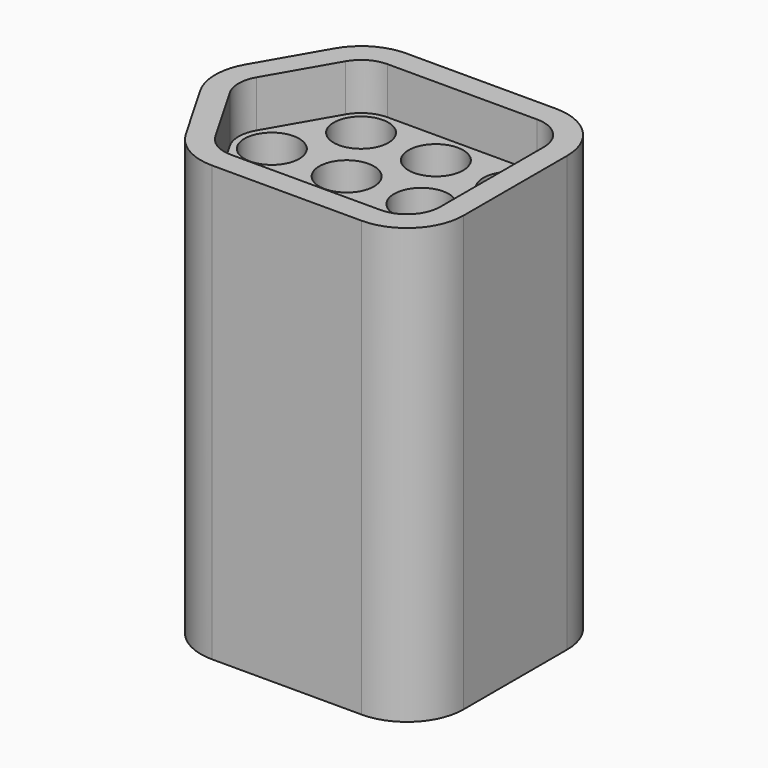
from build123d import *

# Parameters (mm, degrees)
F0_R     = 0.585
F1_DEPTH = 9.3
F2_DEPTH = 1
F3_DEPTH = 8.3
F4_R     = 0.45
F5_DEPTH = 9.301


# Not quite as in the source:
# - a feature names something its author has since deleted; it is built from what else it names


with BuildPart() as f1:
    # F0 (on Top) → F1 (new body)
    with BuildSketch(Plane.XY):
        with BuildLine():
            Line((0, 1.21), (-3.2, 1.21))
            ThreePointArc((-3.2, 1.21), (-3.8050588257, 1.0478567734), (-4.2479586591, 0.6048823429))
            Line((-4.2479586591, 0.6048823429), (-5.0479586591, -0.7811176571))
            ThreePointArc((-5.0479586591, -0.7811176571), (-5.21, -1.386), (-5.0479586591, -1.9908823429))
            Line((-5.0479586591, -1.9908823429), (-4.2479586591, -3.3768823429))
            ThreePointArc((-4.2479586591, -3.3768823429), (-3.8050588257, -3.8198567734), (-3.2, -3.982))
            Line((-3.2, -3.982), (0, -3.982))
            ThreePointArc((0, -3.982), (0.8555992052, -3.6275992052), (1.21, -2.772))
            Line((1.21, -2.772), (1.21, 0))
            ThreePointArc((1.21, 0), (0.8555992052, 0.8555992052), (0, 1.21))
        make_face()
        with BuildLine():
            ThreePointArc((-3.8149178909, 0.3549309616), (-3.5550345175, 0.6148581067), (-3.2, 0.71))
            Line((-3.2, 0.71), (0, 0.71))
            ThreePointArc((0, 0.71), (0.5020458146, 0.5020458146), (0.71, 0))
            Line((0.71, 0), (0.71, -2.772))
            ThreePointArc((0.71, -2.772), (0.5020458146, -3.2740458146), (0, -3.482))
            Line((0, -3.482), (-3.2, -3.482))
            ThreePointArc((-3.2, -3.482), (-3.5550345175, -3.3868581067), (-3.8149178909, -3.1269309616))
            Line((-3.8149178909, -3.1269309616), (-4.6149178909, -1.7409309616))
            ThreePointArc((-4.6149178909, -1.7409309616), (-4.71, -1.386), (-4.6149178909, -1.0310690384))
            Line((-4.6149178909, -1.0310690384), (-3.8149178909, 0.3549309616))
        make_face(mode=Mode.SUBTRACT)
        with BuildLine():
            Line((0, 0.71), (-3.2, 0.71))
            ThreePointArc((-3.2, 0.71), (-3.5550345175, 0.6148581067), (-3.8149178909, 0.3549309616))
            Line((-3.8149178909, 0.3549309616), (-4.6149178909, -1.0310690384))
            ThreePointArc((-4.6149178909, -1.0310690384), (-4.71, -1.386), (-4.6149178909, -1.7409309616))
            Line((-4.6149178909, -1.7409309616), (-3.8149178909, -3.1269309616))
            ThreePointArc((-3.8149178909, -3.1269309616), (-3.5550345175, -3.3868581067), (-3.2, -3.482))
            Line((-3.2, -3.482), (0, -3.482))
            ThreePointArc((0, -3.482), (0.5020458146, -3.2740458146), (0.71, -2.772))
            Line((0.71, -2.772), (0.71, 0))
            ThreePointArc((0.71, 0), (0.5020458146, 0.5020458146), (0, 0.71))
        make_face()
        with Locations((-3.2, -2.772)):
            Circle(F0_R, mode=Mode.SUBTRACT)
        with Locations((-4, -1.386)):
            Circle(F0_R, mode=Mode.SUBTRACT)
        with Locations((-2.4, -1.386)):
            Circle(F0_R, mode=Mode.SUBTRACT)
        with Locations((-1.6, -2.772)):
            Circle(F0_R, mode=Mode.SUBTRACT)
        with Locations((0, -2.772)):
            Circle(F0_R, mode=Mode.SUBTRACT)
        with Locations((-0.8, -1.386)):
            Circle(F0_R, mode=Mode.SUBTRACT)
        with Locations((-3.2, 0)):
            Circle(F0_R, mode=Mode.SUBTRACT)
        with Locations((-1.6, 0)):
            Circle(F0_R, mode=Mode.SUBTRACT)
        Circle(F0_R, mode=Mode.SUBTRACT)
        with Locations((-4, -1.386)):
            Circle(F0_R)
        with Locations((-3.2, 0)):
            Circle(F0_R)
        with Locations((-1.6, 0)):
            Circle(F0_R)
        with Locations((-2.4, -1.386)):
            Circle(F0_R)
        with Locations((-3.2, -2.772)):
            Circle(F0_R)
        with Locations((-1.6, -2.772)):
            Circle(F0_R)
        with Locations((-0.8, -1.386)):
            Circle(F0_R)
        Circle(F0_R)
        with Locations((0, -2.772)):
            Circle(F0_R)
    extrude(amount=-F1_DEPTH)

    # F0 (on Top) → F2 (cut)
    with BuildSketch(Plane.XY):
        with BuildLine():
            Line((0, 0.71), (-3.2, 0.71))
            ThreePointArc((-3.2, 0.71), (-3.5550345175, 0.6148581067), (-3.8149178909, 0.3549309616))
            Line((-3.8149178909, 0.3549309616), (-4.6149178909, -1.0310690384))
            ThreePointArc((-4.6149178909, -1.0310690384), (-4.71, -1.386), (-4.6149178909, -1.7409309616))
            Line((-4.6149178909, -1.7409309616), (-3.8149178909, -3.1269309616))
            ThreePointArc((-3.8149178909, -3.1269309616), (-3.5550345175, -3.3868581067), (-3.2, -3.482))
            Line((-3.2, -3.482), (0, -3.482))
            ThreePointArc((0, -3.482), (0.5020458146, -3.2740458146), (0.71, -2.772))
            Line((0.71, -2.772), (0.71, 0))
            ThreePointArc((0.71, 0), (0.5020458146, 0.5020458146), (0, 0.71))
        make_face()
        with Locations((-3.2, -2.772)):
            Circle(F0_R, mode=Mode.SUBTRACT)
        with Locations((-4, -1.386)):
            Circle(F0_R, mode=Mode.SUBTRACT)
        with Locations((-2.4, -1.386)):
            Circle(F0_R, mode=Mode.SUBTRACT)
        with Locations((-1.6, -2.772)):
            Circle(F0_R, mode=Mode.SUBTRACT)
        with Locations((0, -2.772)):
            Circle(F0_R, mode=Mode.SUBTRACT)
        with Locations((-0.8, -1.386)):
            Circle(F0_R, mode=Mode.SUBTRACT)
        with Locations((-3.2, 0)):
            Circle(F0_R, mode=Mode.SUBTRACT)
        with Locations((-1.6, 0)):
            Circle(F0_R, mode=Mode.SUBTRACT)
        Circle(F0_R, mode=Mode.SUBTRACT)
        Circle(F0_R)
        with Locations((-0.8, -1.386)):
            Circle(F0_R)
        with Locations((0, -2.772)):
            Circle(F0_R)
        with Locations((-4, -1.386)):
            Circle(F0_R)
        with Locations((-2.4, -1.386)):
            Circle(F0_R)
        with Locations((-3.2, 0)):
            Circle(F0_R)
        with Locations((-1.6, 0)):
            Circle(F0_R)
        with Locations((-1.6, -2.772)):
            Circle(F0_R)
        with Locations((-3.2, -2.772)):
            Circle(F0_R)
    extrude(amount=-F2_DEPTH, mode=Mode.SUBTRACT)

    # F0 (on Top) → F3 (cut)
    with BuildSketch(Plane.XY):
        with Locations((-0.8, -1.386)):
            Circle(F0_R)
        Circle(F0_R)
        with Locations((0, -2.772)):
            Circle(F0_R)
        with Locations((-1.6, -2.772)):
            Circle(F0_R)
        with Locations((-3.2, -2.772)):
            Circle(F0_R)
        with Locations((-2.4, -1.386)):
            Circle(F0_R)
        with Locations((-1.6, 0)):
            Circle(F0_R)
        with Locations((-3.2, 0)):
            Circle(F0_R)
        with Locations((-4, -1.386)):
            Circle(F0_R)
    extrude(amount=-F3_DEPTH, mode=Mode.SUBTRACT)

    # F4 (on Top) → F5 (cut, through all)
    with BuildSketch(Plane.XY):
        with Locations((-3.2, 0)):
            Circle(F4_R)
        with Locations((-1.6, 0)):
            Circle(F4_R)
        Circle(F4_R)
        with Locations((-0.8, -1.386)):
            Circle(F4_R)
        with Locations((-2.4, -1.386)):
            Circle(F4_R)
        with Locations((-4, -1.386)):
            Circle(F4_R)
        with Locations((-3.2, -2.772)):
            Circle(F4_R)
        with Locations((-1.6, -2.772)):
            Circle(F4_R)
        with Locations((0, -2.772)):
            Circle(F4_R)
    extrude(amount=-F5_DEPTH, mode=Mode.SUBTRACT)


solid = f1.part
